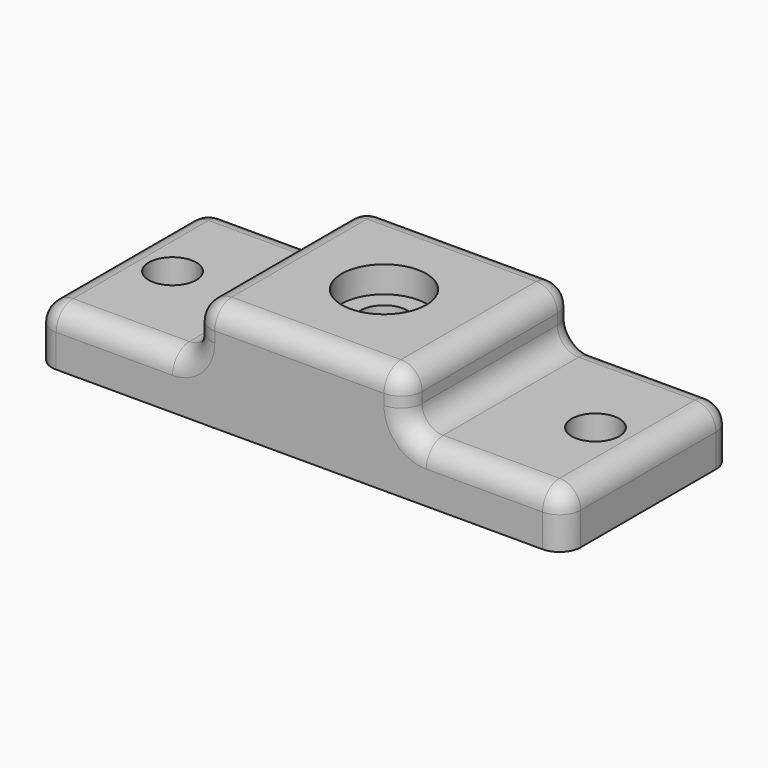
from build123d import *

# Parameters (mm, degrees)
F0_W     = 50
F0_H     = 20
F0_R     = 2.25
F0_R_2   = 4
F0_R_3   = 3
F1_DEPTH = 5.1
F2_W     = 20
F2_H     = 20
F2_R     = 3
F2_R_2   = 2.25
F3_DEPTH = 2.5
F4_W     = 20
F4_H     = 20
F4_R     = 4
F5_DEPTH = 2.5
F6_R     = 2


# Not quite as in the source:
# - a feature names something its author has since deleted; it is built from what else it names


with BuildPart() as f1:
    # F0 (on Top) → F1 (new body)
    with BuildSketch(Plane.XY):
        Rectangle(F0_W, F0_H)
        with Locations((-20, 0)):
            Circle(F0_R, mode=Mode.SUBTRACT)
        Circle(F0_R_2, mode=Mode.SUBTRACT)
        with Locations((20, 0)):
            Circle(F0_R, mode=Mode.SUBTRACT)
        Circle(F0_R_2)
        Circle(F0_R_3, mode=Mode.SUBTRACT)
    extrude(amount=F1_DEPTH)

    # F2 (on face) → F3 (join)
    with BuildSketch(Plane.XY.offset(5.1)):
        Rectangle(F2_W, F2_H)
        Circle(F2_R, mode=Mode.SUBTRACT)
        Circle(F2_R)
        Circle(F2_R_2, mode=Mode.SUBTRACT)
    extrude(amount=F3_DEPTH)

    # F4 (on face) → F5 (join)
    with BuildSketch(Plane.XY.offset(7.6)):
        Rectangle(F4_W, F4_H)
        Circle(F4_R, mode=Mode.SUBTRACT)
    extrude(amount=F5_DEPTH)

    # F6
    f6_edges = [f1.edges().sort_by_distance(p)[0] for p in [
        (-25, -10, 2.55),
        (25, -10, 2.55),
        (25, 10, 2.55),
        (25, 0, 5.1),
        (17.5, -10, 5.1),
        (17.5, 10, 5.1),
        (-17.5, -10, 5.1),
        (-25, 0, 5.1),
        (-17.5, 10, 5.1),
        (-25, 10, 2.55),
        (10, -10, 7.6),
        (10, 10, 7.6),
        (-10, -10, 7.6),
        (-10, 10, 7.6),
        (10, 0, 5.1),
        (-10, 0, 5.1),
        (0, -10, 10.1),
        (-10, 0, 10.1),
        (0, 10, 10.1),
        (10, 0, 10.1),
    ]]
    fillet(f6_edges, radius=F6_R)


solid = f1.part
